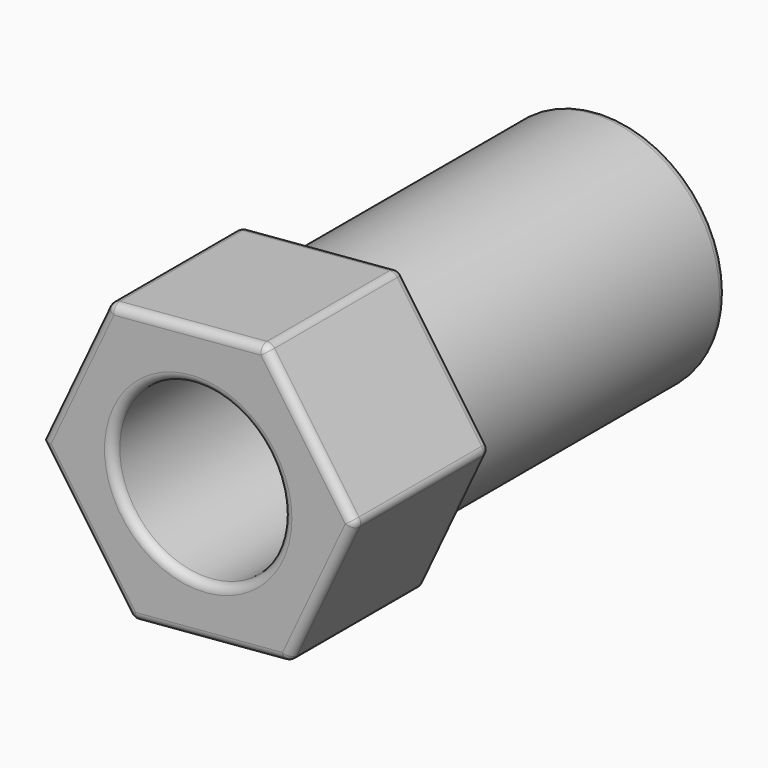
from build123d import *

# Parameters (mm, degrees)
F0_R     = 3.5
F0_R_2   = 2.5
F1_DEPTH = 10
F2_START = 10
F2_DEPTH = 5
F3_R     = 0.24999


# Not quite as in the source:
# - a fillet or chamfer is up to 0.001 mm smaller than in the source, because OpenCascade refuses the exact size


with BuildPart() as f1:
    # F0 (on Front) → F1 (new body)
    with BuildSketch(Plane.XZ):
        Circle(F0_R)
        Circle(F0_R_2, mode=Mode.SUBTRACT)
    extrude(amount=F1_DEPTH)

    # F0 (on Front) → F2 (join)
    with BuildSketch(Plane.XZ.offset(F2_START)):
        Polygon((2.6409240726, -3.78930777), (4.6020988279, 0.3924534514), (1.9611747553, 4.1817612214), (-2.6409240726, 3.78930777), (-4.6020988279, -0.3924534514), (-1.9611747553, -4.1817612214), align=None)
        Circle(F0_R, mode=Mode.SUBTRACT)
        Circle(F0_R)
        Circle(F0_R_2, mode=Mode.SUBTRACT)
    extrude(amount=F2_DEPTH)

    # F3 (radius 0.25 in the source; OpenCascade refuses exactly that, so slightly less here)
    f3_edges = [f1.edges().sort_by_distance(p)[0] for p in [
        (-2.5, -15, 0),
        (-0.339875, -15, 3.985534),
        (-0.339875, -10, 3.985534),
        (1.961175, -12.5, 4.181761),
        (-3.5, 0, 0),
        (-2.640924, -12.5, 3.789308),
        (-3.621511, -15, 1.698427),
        (-3.281637, -15, -2.287107),
        (-3.621511, -10, 1.698427),
        (-3.281637, -10, -2.287107),
        (-1.961175, -12.5, -4.181761),
        (0.339875, -10, -3.985534),
        (2.640924, -12.5, -3.789308),
        (0.339875, -15, -3.985534),
        (3.621511, -15, -1.698427),
        (3.281637, -15, 2.287107),
        (4.602099, -12.5, 0.392453),
        (3.621511, -10, -1.698427),
        (3.281637, -10, 2.287107),
        (-3.5, -10, 0),
        (-2.5, 0, 0),
    ]]
    fillet(f3_edges, radius=F3_R)


solid = f1.part
